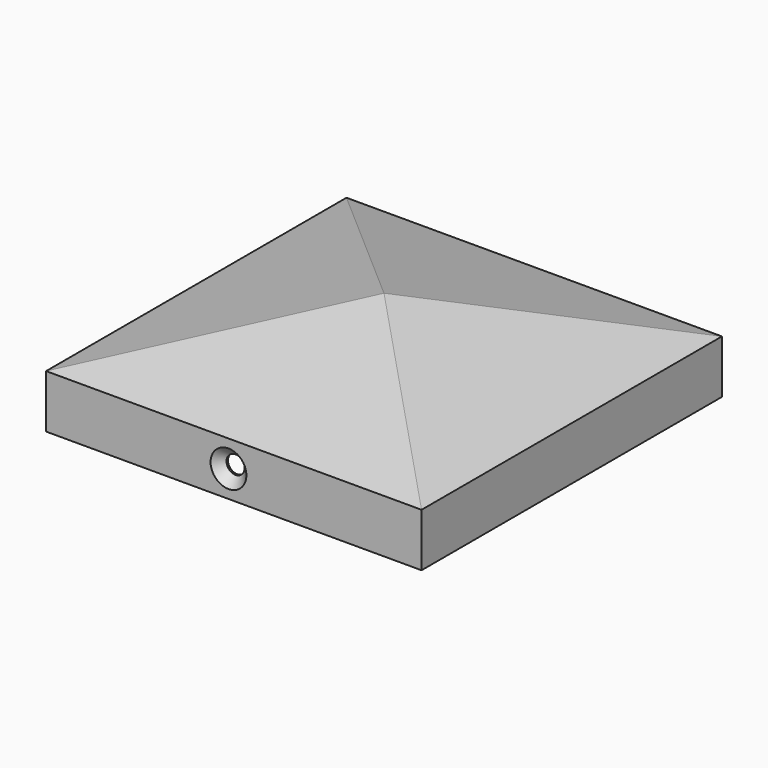
from build123d import *

# Parameters (mm, degrees)
F0_W                 = 70.5
F0_H                 = 70.5
F1_DEPTH             = 10
F2_W                 = 70.5
F2_H                 = 70.5
F3_DEPTH             = 10
F4_SIZE2             = 9.99999
F4_SIZE              = 35.24999
F5_W                 = 66.5
F5_H                 = 66.5
F6_DEPTH             = 8
F9_D                 = 3.4
F9_DEPTH             = 12
F9_CSINK_D           = 6.72
F9_CSINK_ANGLE       = 90
F9_TIP               = 1.0214630523
F9_ON_F8_D           = 3.4
F9_ON_F8_DEPTH       = 12
F9_ON_F8_CSINK_D     = 6.72
F9_ON_F8_CSINK_ANGLE = 90
F9_ON_F8_TIP         = 1.0214630523


# Not quite as in the source:
# - a fillet or chamfer is up to 0.001 mm smaller than in the source, because OpenCascade refuses the exact size


with BuildPart() as f1:
    # F0 (on Top) → F1 (new body)
    with BuildSketch(Plane.XY):
        with Locations((35.25, 35.25)):
            Rectangle(F0_W, F0_H)
    extrude(amount=F1_DEPTH)

    # F2 (on face) → F3 (join)
    with BuildSketch(Plane.XY.offset(10)):
        with Locations((35.25, 35.25)):
            Rectangle(F2_W, F2_H)
    extrude(amount=F3_DEPTH)

    # F4 (size 35.25 and 10 in the source; OpenCascade refuses exactly that, so slightly less here)
    f4_edges = [f1.edges().sort_by_distance(p)[0] for p in [
        (35.25, 70.5, 20),
        (0, 35.25, 20),
        (35.25, 0, 20),
        (70.5, 35.25, 20),
    ]]
    f4_side = f1.faces().sort_by_distance((35.25, 35.25, 20))[0]
    chamfer(f4_edges, length=F4_SIZE, length2=F4_SIZE2, reference=f4_side)

    # F5 (on face) → F6 (cut)
    with BuildSketch(Plane(origin=(0, 0, 0), x_dir=(1, 0, 0), z_dir=(0, 0, -1))):
        with Locations((35.25, -35.25)):
            Rectangle(F5_W, F5_H)
    extrude(amount=-F6_DEPTH, mode=Mode.SUBTRACT)

    # F9
    with Locations(Plane.XZ):
        with Locations((34.25, 5)):
            CounterSinkHole(F9_D / 2, F9_CSINK_D / 2, depth=F9_DEPTH, counter_sink_angle=F9_CSINK_ANGLE)
            with Locations((0, 0, -(F9_DEPTH + F9_TIP / 2))):  # 118° drill point
                Cone(0, F9_D / 2, F9_TIP, mode=Mode.SUBTRACT)

    # F9 on F8
    with Locations(Plane(origin=(0, 70.5, 0), x_dir=(-1, 0, 0), z_dir=(0, 1, 0))):
        with Locations((-34.25, 5)):
            CounterSinkHole(F9_ON_F8_D / 2, F9_ON_F8_CSINK_D / 2, depth=F9_ON_F8_DEPTH, counter_sink_angle=F9_ON_F8_CSINK_ANGLE)
            with Locations((0, 0, -(F9_ON_F8_DEPTH + F9_ON_F8_TIP / 2))):  # 118° drill point
                Cone(0, F9_ON_F8_D / 2, F9_ON_F8_TIP, mode=Mode.SUBTRACT)


solid = f1.part
